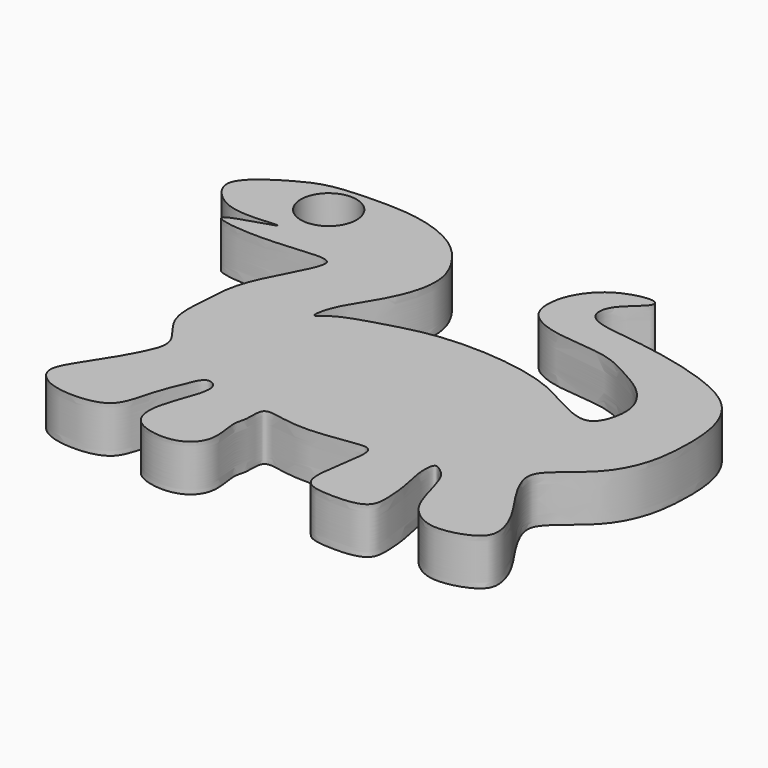
from build123d import *

# Parameters (mm, degrees)
F1_DEPTH = 5
F2_R     = 2.9970440669
F3_DEPTH = 5


with BuildPart() as f1:
    # F0 (on Top) → F1 (new body)
    with BuildSketch(Plane.XY):
        with BuildLine():
            add(Edge.make_bspline(
                [(-56.4708225429, 50.6098866463), (-55.246993339, 51.2948686943), (-53.4114845302, 52.0860943781), (-48.3322544899, 52.28495809), (-43.9833023684, 52.1084314009), (-40.0035494073, 50.7178069938), (-37.4487411719, 48.5640558527), (-35.3931712193, 45.1626824353), (-35.7399463726, 41.4480291005), (-37.5613174183, 37.7572901602), (-39.6093979914, 34.8792265962), (-40.0592281403, 32.045782415), (-38.6069683601, 33.7527622683), (-34.4043488924, 34.9921342387), (-29.6228781061, 36.3815501843), (-23.0264638702, 36.4397302251), (-16.9769467748, 35.2079915002), (-13.6179493656, 33.1269104546), (-9.7783442876, 31.3364832835), (-8.4623735877, 33.6944284071), (-8.2334306142, 36.5633701747), (-10.171382727, 39.2032002189), (-12.7967057814, 40.6226204446), (-16.1529522793, 42.5758965002), (-21.912035404, 42.4847663705), (-25.7115813221, 44.2660060372), (-25.8738141563, 47.2951154583), (-24.9855363581, 49.640286688), (-22.7727024941, 52.0547757452), (-19.0469419629, 52.866419458), (-18.4985286074, 51.6499491482), (-21.6309266481, 49.6977701616), (-21.7047195248, 46.4528769607), (-16.5494031926, 45.9788942099), (-12.1523322258, 45.2452484045), (-7.9967322712, 44.2095792657), (-2.9363293971, 42.1297142324), (-0.6574527286, 37.9340773754), (-0.5983028567, 32.7963713646), (-1.0939654447, 29.1056443277), (-3.0551951111, 25.1251122645), (-7.5850255392, 22.285914177), (-7.5233184338, 19.9102765324), (-5.6069622415, 16.7764462133), (-3.7506047108, 14.2105071841), (-2.8159136484, 11.2341858781), (-4.0378220227, 9.5799361051), (-7.8857032758, 8.4659692933), (-10.4427919567, 9.8160050889), (-11.9211030647, 11.8752607054), (-12.8224027165, 16.3087429926), (-13.8827112132, 17.2212097626), (-15.002976695, 18.044370057), (-15.1476484626, 15.7703964263), (-14.4330947016, 13.2556050895), (-14.2261290092, 10.7863623386), (-14.2653924997, 8.0883942098), (-18.4282667818, 7.8576499568), (-21.5917860435, 8.2931009891), (-21.3828213995, 11.6898190881), (-20.6190903943, 15.3673990447), (-20.9862152931, 16.7741469409), (-22.8313035793, 16.6510085775), (-27.0468531055, 15.925459061), (-30.0209952221, 16.2560950496), (-32.6943728538, 16.9265327947), (-32.3137610334, 14.3379326524), (-33.0173094312, 13.1219082384), (-31.9880589789, 9.6397639726), (-34.4368083766, 6.9822979013), (-39.6289784986, 7.8061806875), (-40.0405379165, 11.2570529681), (-38.7553976092, 14.3953489716), (-37.9061515698, 17.3666518345), (-39.669552001, 18.1906842798), (-40.5335366688, 16.084889518), (-41.8428180441, 12.9013974083), (-42.4734549133, 9.1895834309), (-46.2475673062, 8.4343126748), (-49.7477408606, 8.9616695559), (-51.5698969354, 11.1027824253), (-49.4147782768, 14.2609859729), (-46.5948444748, 18.8192462069), (-45.8207418054, 21.6914728702), (-49.1650034274, 24.5936831002), (-48.5695540252, 29.5715685553), (-48.5599271528, 33.8381510764), (-44.2621667188, 40.4461433142), (-45.6211048272, 41.4376463183), (-48.7817412171, 41.0364074128), (-54.3435769441, 40.7799409294), (-57.6111955909, 41.5337198198), (-55.9111334334, 42.4015139195), (-50.374262171, 43.9080867979), (-56.2487753209, 43.0814227509), (-59.1928878579, 44.185076854), (-61.5971859639, 47.4562272289), (-57.9781625312, 49.7662224904), (-56.4708225429, 50.6098866463)],
                knots=[0, 0, 0, 0, 0.0108111921, 0.0235970589, 0.0359285092, 0.0476178726, 0.0581879196, 0.0694452178, 0.0804132835, 0.092172484, 0.1036008406, 0.111391292, 0.1178148466, 0.1300769625, 0.1432483904, 0.1581874966, 0.1724989233, 0.1843624384, 0.1952930897, 0.2036152116, 0.2133340897, 0.2234906162, 0.2334500716, 0.2447685498, 0.2587772994, 0.2700345976, 0.2793627338, 0.2884388069, 0.2990859805, 0.3097584944, 0.3144263331, 0.3250735087, 0.333862551, 0.3461633282, 0.3587906084, 0.3708338324, 0.3841219111, 0.3964751285, 0.4094823152, 0.4206466662, 0.432840509, 0.4458028319, 0.4539300343, 0.4648996521, 0.4755923109, 0.4853067269, 0.4930225368, 0.5042912948, 0.5137671498, 0.5230674299, 0.5352113068, 0.5421913626, 0.5474996266, 0.5549180203, 0.564713993, 0.5740015268, 0.5824144605, 0.5936008045, 0.6032108726, 0.6130927833, 0.6246132478, 0.6306289934, 0.6378107459, 0.6499317049, 0.6605104068, 0.6686223181, 0.6765925549, 0.6836202602, 0.6940542789, 0.7042127621, 0.7163851045, 0.7261372463, 0.7371926651, 0.7467981164, 0.7529936357, 0.7608608435, 0.7720369435, 0.7827245763, 0.7934021386, 0.8043343539, 0.8127916118, 0.8235849438, 0.8373121417, 0.8466175042, 0.8579570939, 0.8703962515, 0.8831536361, 0.8985874798, 0.9041022744, 0.9142529352, 0.9287053813, 0.9374823377, 0.9440907699, 0.9552241123, 0.9657889558, 0.9769222982, 0.9866843003, 1, 1, 1, 1], degree=3))
        make_face()
    extrude(amount=F1_DEPTH)

    # F2 (on face) → F3 (cut)
    with BuildSketch(Plane.XY.offset(5)):
        with Locations((-50.8610270917, 48.425167799)):
            Circle(F2_R)
    extrude(amount=-F3_DEPTH, mode=Mode.SUBTRACT)


solid = f1.part
